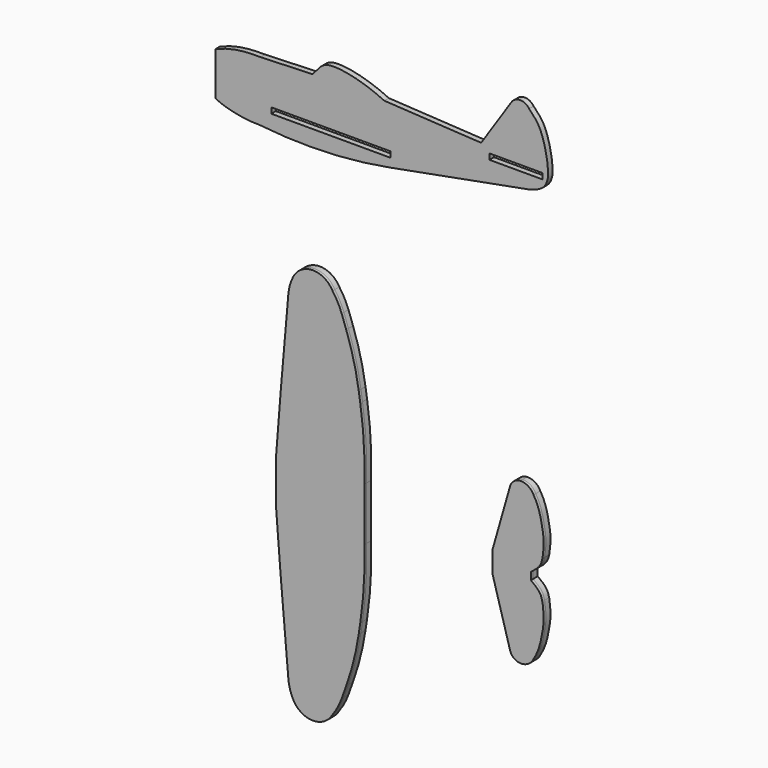
from build123d import *

# Parameters (mm, degrees)
F1_DEPTH = 3.175
F2_W     = 66.7287356216
F2_H     = 3.175
F2_W_2   = 29.7339134365
F3_DEPTH = 3.1760001
F4_DEPTH = 1.5875


# Not quite as in the source:
# - a feature names something its author has since deleted; it is built from what else it names


with BuildPart() as f1:
    # F0 (on Front) → F1 (new body)
    with BuildSketch(Plane.XZ):
        with BuildLine():
            add(Edge.make_bspline(
                [(-217.2774374485, 316.1117434502), (-208.2704752684, 320.0652301311), (-200.7178515196, 320.5276429653), (-191.9366121292, 320.4519748688)],
                knots=[0, 0, 0, 0, 25.7098237378, 25.7098237378, 25.7098237378, 25.7098237378], degree=3))
            Line((-217.2774374485, 316.1117434502), (-217.2774374485, 292.066693306))
            add(Edge.make_bspline(
                [(-217.2774374485, 292.066693306), (-211.6587013006, 288.8643443584), (-200.9846866131, 286.8784666061), (-192.2965347767, 286.8784666061)],
                knots=[0, 0, 0, 0, 25.5139803752, 25.5139803752, 25.5139803752, 25.5139803752], degree=3))
            ThreePointArc((-192.2965347767, 286.8784666061), (-155.9543345014, 285.583535578), (-119.8125630617, 289.6090447903))
            Line((-119.8125630617, 289.6090447903), (-41.8674536049, 304.1306734085))
            add(Edge.make_bspline(
                [(-41.8674536049, 343.847900629), (-39.9035527612, 341.8708754749), (-35.6939266118, 337.6331173347), (-32.5058142024, 326.5151935972), (-31.3577674671, 319.4689798911), (-30.9266074047, 312.9104055483), (-33.7005376, 306.5830268044), (-39.0145912431, 304.9873280743), (-41.8674536049, 304.1306734085)],
                knots=[0, 0, 0, 0, 0.1741781632, 0.3733513087, 0.5334575375, 0.6824963743, 0.8295474219, 1, 1, 1, 1], degree=3))
            ThreePointArc((-41.8674536049, 343.847900629), (-46.8321088701, 346.5121071855), (-51.7967641354, 343.847900629))
            add(Edge.make_bspline(
                [(-68.6765983701, 318.4040486813), (-63.0499869585, 326.8853326639), (-57.4233755469, 335.3666166464), (-51.7967641354, 343.847900629)],
                knots=[0, 0, 0, 0, 30.5338894629, 30.5338894629, 30.5338894629, 30.5338894629], degree=3))
            add(Edge.make_bspline(
                [(-122.7908893077, 321.5055249581), (-96.9993255664, 319.9876210494), (-69.4583634176, 318.3667602704), (-68.7232901316, 318.4018215907), (-68.6765983701, 318.4040486813)],
                knots=[0, 0, 0, 0, 0.9364801274, 1, 1, 1, 1], degree=3))
            add(Edge.make_bspline(
                [(-163.0044796912, 321.5055249581), (-158.9115120044, 326.1343460077), (-155.7485347114, 331.5570526506), (-135.0788772106, 327.3404538631), (-122.7908893077, 321.5055249581)],
                knots=[0, 0, 0, 0, 0.3748449886, 1, 1, 1, 1], degree=3))
            add(Edge.make_bspline(
                [(-191.9366121292, 320.4519748688), (-182.2927643855, 320.8036422729), (-172.6483274348, 321.1538575539), (-163.0044796912, 321.5055249581)],
                knots=[0, 0, 0, 0, 28.9513083505, 28.9513083505, 28.9513083505, 28.9513083505], degree=3))
        make_face()
    extrude(amount=F1_DEPTH)

    # F2 (on Front) → F3 (cut, through all)
    with BuildSketch(Plane.XZ):
        with Locations((-152.6276346764, 296.1412173271)):
            Rectangle(F2_W, F2_H)
        with Locations((-49.1691168621, 313.1201070309)):
            Rectangle(F2_W_2, F2_H)
    extrude(amount=F3_DEPTH, mode=Mode.SUBTRACT)


with BuildPart() as f1b:
    # F0 (on Front) → F1, piece 2 (new body)
    with BuildSketch(Plane.XZ):
        with BuildLine():
            Line((-179.445758462, 160.8685404062), (-181.9537132978, 129.0372312069))
            Line((-181.9537132978, 129.0372312069), (-181.9537132978, 115.3391599655))
            Line((-181.9537132978, 115.3391599655), (-181.9537132978, 101.6410887241))
            Line((-181.9537132978, 101.6410887241), (-179.445758462, 69.8097795248))
            Line((-179.445758462, 69.8097795248), (-175.1670092344, 20.6041038036))
            ThreePointArc((-175.1670092344, 20.6041038036), (-174.2360127213, 15.7024883336), (-172.3408847108, 11.087179184))
            ThreePointArc((-172.3408847108, 11.087179184), (-161.4089235194, 4.5326941653), (-150.476962328, 11.087179184))
            ThreePointArc((-150.476962328, 11.087179184), (-147.5813077332, 15.658789231), (-145.3839689493, 20.6041038036))
            Line((-145.3839689493, 20.6041038036), (-142.820417881, 27.7401655912))
            ThreePointArc((-142.820417881, 27.7401655912), (-138.6554382828, 41.4030806133), (-135.8470420761, 55.4079088057))
            Line((-135.8470420761, 55.4079088057), (-134.9724531174, 61.2375587225))
            ThreePointArc((-134.9724531174, 61.2375587225), (-132.9361148448, 80.8054911513), (-132.6754838228, 100.4773676395))
            Line((-132.6754838228, 100.4773676395), (-132.6754838228, 115.3391599655))
            Line((-132.6754838228, 115.3391599655), (-132.6754838228, 130.2009522915))
            ThreePointArc((-132.6754838228, 130.2009522915), (-132.9361148448, 149.8728287797), (-134.9724531174, 169.4407612085))
            Line((-134.9724531174, 169.4407612085), (-135.8470420761, 175.2704111254))
            ThreePointArc((-135.8470420761, 175.2704111254), (-138.6554382828, 189.2752393178), (-142.820417881, 202.9381543398))
            Line((-142.820417881, 202.9381543398), (-145.3839689493, 210.0742161274))
            ThreePointArc((-145.3839689493, 210.0742161274), (-147.5813077332, 215.0195307001), (-150.476962328, 219.5911407471))
            ThreePointArc((-150.476962328, 219.5911407471), (-161.4089235194, 226.1456257657), (-172.3408847108, 219.5911407471))
            ThreePointArc((-172.3408847108, 219.5911407471), (-174.2360127213, 214.9758315974), (-175.1670092344, 210.0742161274))
            Line((-175.1670092344, 210.0742161274), (-179.445758462, 160.8685404062))
        make_face()
    extrude(amount=F1_DEPTH)


with BuildPart() as f1c:
    # F0 (on Front) → F1, piece 3 (new body)
    with BuildSketch(Plane.XZ):
        with BuildLine():
            Line((-61.1366257071, 121.0409328341), (-61.1366257071, 115.3391599655))
            Line((-61.1366257071, 115.3391599655), (-61.1366257071, 109.6373870969))
            Line((-61.1366257071, 109.6373870969), (-51.2456595898, 74.9716758728))
            ThreePointArc((-51.2456595898, 74.9716758728), (-49.1167179542, 71.795143879), (-45.5316118896, 70.4648196697))
            ThreePointArc((-45.5316118896, 70.4648196697), (-41.1453075948, 71.5941314621), (-38.1274931133, 74.9716758728))
            add(Edge.make_bspline(
                [(-38.1274931133, 74.9716758728), (-37.7114533868, 75.6467806233), (-36.6980818799, 77.2960212626), (-34.5607015396, 82.3765499704), (-33.29842215, 89.0787746733), (-32.3154011086, 94.6055276867), (-32.4336381536, 99.4259350363), (-33.0247754512, 104.611924583), (-33.218242228, 104.8295795918)],
                knots=[0, 0, 0, 0, 0.1126820004, 0.2760413664, 0.4612237316, 0.6245387092, 0.789371414, 0.9424801543, 0.9424801543, 0.9424801543, 0.9424801543], degree=3))
            add(Edge.make_bspline(
                [(-33.218242228, 104.8295795918), (-33.4641640419, 105.9295439447), (-33.9617464288, 108.1551410958), (-36.4350424059, 110.8177781387), (-38.2271971963, 112.2007073582), (-39.1778436897, 112.9094674542), (-39.617408067, 113.2371872663)],
                knots=[0, 0, 0, 0, 0.281901241, 0.5703808466, 0.801350684, 1, 1, 1, 1], degree=3))
            Line((-39.617408067, 113.2371872663), (-39.617408067, 115.3391599655))
            Line((-39.617408067, 115.3391599655), (-39.617408067, 117.4411326647))
            add(Edge.make_bspline(
                [(-33.218242228, 125.8487403393), (-33.4641640419, 124.7487759864), (-33.9617464288, 122.5231788353), (-36.4350424059, 119.8605417924), (-38.2271971963, 118.4776125728), (-39.1778436897, 117.7688524769), (-39.617408067, 117.4411326647)],
                knots=[0, 0, 0, 0, 0.281901241, 0.5703808466, 0.801350684, 1, 1, 1, 1], degree=3))
            add(Edge.make_bspline(
                [(-38.1274931133, 155.7066440582), (-37.7114533868, 155.0315393077), (-36.6980818799, 153.3822986684), (-34.5607015396, 148.3017699606), (-33.29842215, 141.5995452578), (-32.3154011086, 136.0727922443), (-32.4336381536, 131.2523848947), (-33.0247754512, 126.066395348), (-33.218242228, 125.8487403393)],
                knots=[0, 0, 0, 0, 0.1126820004, 0.2760413664, 0.4612237316, 0.6245387092, 0.789371414, 0.9424801543, 0.9424801543, 0.9424801543, 0.9424801543], degree=3))
            ThreePointArc((-38.1274931133, 155.7066440582), (-41.1453075948, 159.0841884689), (-45.5316118896, 160.2135002613))
            ThreePointArc((-45.5316118896, 160.2135002613), (-49.1167179542, 158.8831760521), (-51.2456595898, 155.7066440582))
            Line((-51.2456595898, 155.7066440582), (-61.1366257071, 121.0409328341))
        make_face()
    extrude(amount=F1_DEPTH)


with BuildPart() as f4:
    # F4 (new): a face of the model
    f4_faces = [f1b.part.faces().sort_by_distance(p)[0] for p in [
        (-157.6168541364, -3.175, 115.3391599655),
    ]]
    extrude(f4_faces, amount=F4_DEPTH)


with BuildPart() as f4b:
    # F4#2 (new): a face of the model
    f4_2_faces = [f1c.part.faces().sort_by_distance(p)[0] for p in [
        (-45.7775339149, -3.175, 115.3391599655),
    ]]
    extrude(f4_2_faces, amount=F4_DEPTH)


solid = Compound([f1.part, f1b.part, f1c.part, f4.part, f4b.part])
